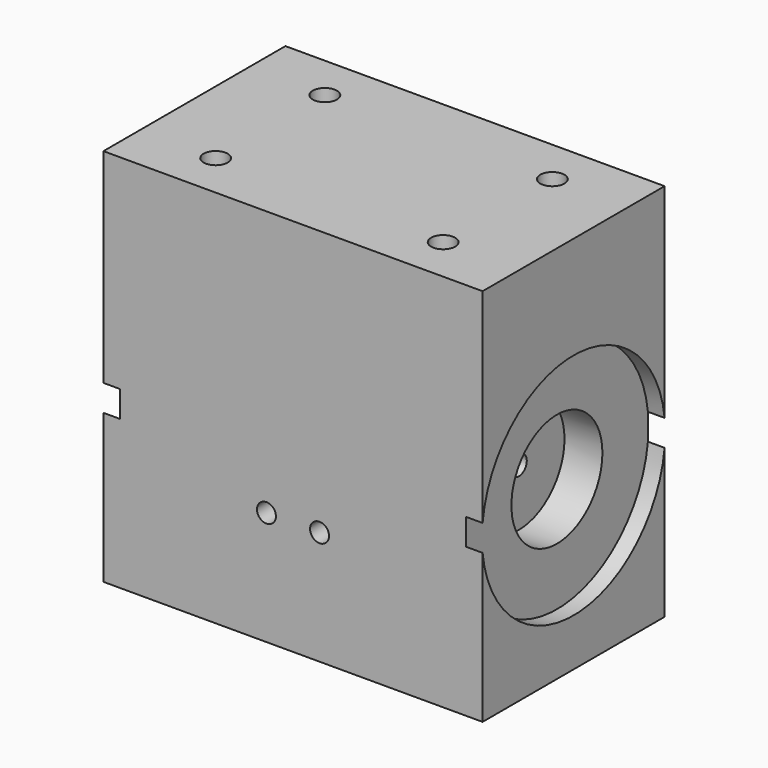
from build123d import *
from build123d import SkipClean  # not in build123d's __all__

# Parameters (mm, degrees)
F0_W      = 63.5
F0_H      = 38.1
F0_R      = 2.0193
F1_DEPTH  = 63.5
F2_DEPTH  = 25.4
F3_R      = 2.0193
F4_DEPTH  = 25.4
F5_R      = 1.5875
F6_DEPTH  = 19.05
F7_R      = 1.5875
F8_DEPTH  = 20.32
F9_R      = 1.63195
F10_DEPTH = 63.501
F9_R_2    = 9.525
F11_DEPTH = 9.144
F12_DEPTH = 2.794
F13_R     = 9.525
F13_R_2   = 1.63195
F14_DEPTH = 9.144
F15_DEPTH = 2.794


with BuildPart() as f1:
    # F0 (on Top) → F1 (new body)
    with BuildSketch(Plane.XY):
        Rectangle(F0_W, F0_H)
        with Locations((-24.13, -11.43)):
            Circle(F0_R, mode=Mode.SUBTRACT)
        with Locations((24.13, -11.43)):
            Circle(F0_R, mode=Mode.SUBTRACT)
        with Locations((-24.13, 11.43)):
            Circle(F0_R, mode=Mode.SUBTRACT)
        with Locations((24.13, 11.43)):
            Circle(F0_R, mode=Mode.SUBTRACT)
        with Locations((-24.13, 11.43)):
            Circle(F0_R)
        with Locations((24.13, 11.43)):
            Circle(F0_R)
        with Locations((24.13, -11.43)):
            Circle(F0_R)
        with Locations((-24.13, -11.43)):
            Circle(F0_R)
    extrude(amount=F1_DEPTH)

    # F0 (on Top) → F2 (cut)
    with BuildSketch(Plane.XY):
        with Locations((24.13, 11.43)):
            Circle(F0_R)
        with Locations((24.13, -11.43)):
            Circle(F0_R)
        with Locations((-24.13, 11.43)):
            Circle(F0_R)
        with Locations((-24.13, -11.43)):
            Circle(F0_R)
    extrude(amount=F2_DEPTH, mode=Mode.SUBTRACT)

    # F3 (on face) → F4 (cut)
    with BuildSketch(Plane.XY.offset(63.5)):
        with Locations((-19.05, 11.43)):
            Circle(F3_R)
        with Locations((-19.05, -11.43)):
            Circle(F3_R)
        with Locations((19.05, 11.43)):
            Circle(F3_R)
        with Locations((19.05, -11.43)):
            Circle(F3_R)
    extrude(amount=-F4_DEPTH, mode=Mode.SUBTRACT)

    # F5 (on face) → F6 (cut)
    with BuildSketch(Plane.XY):
        with Locations((-4.445, 0)):
            Circle(F5_R)
        with Locations((4.445, 0)):
            Circle(F5_R)
    extrude(amount=F6_DEPTH, mode=Mode.SUBTRACT)

    # F7 (on face) → F8 (cut)
    with BuildSketch(Plane.XZ.offset(19.05)):
        with Locations((-4.445, 19.05)):
            Circle(F7_R)
        with Locations((4.445, 19.05)):
            Circle(F7_R)
    with SkipClean():  # cleaning this boolean's faces spoils the solid; the shape is the same uncleaned
        extrude(amount=-F8_DEPTH, mode=Mode.SUBTRACT)

    # F9 (on face) → F10 (cut, through all)
    with BuildSketch(Plane.YZ.offset(31.75)):
        with Locations((0, 27.1272)):
            Circle(F9_R)
    with SkipClean():  # cleaning this boolean's faces spoils the solid; the shape is the same uncleaned
        extrude(amount=-F10_DEPTH, mode=Mode.SUBTRACT)

    # F9 (on face) → F11 (cut)
    with BuildSketch(Plane.YZ.offset(31.75)):
        with Locations((0, 27.1272)):
            Circle(F9_R_2)
        with Locations((0, 27.1272)):
            Circle(F9_R, mode=Mode.SUBTRACT)
    with SkipClean():  # cleaning this boolean's faces spoils the solid; the shape is the same uncleaned
        extrude(amount=-F11_DEPTH, mode=Mode.SUBTRACT)

    # F9 (on face) → F12 (cut)
    with BuildSketch(Plane.YZ.offset(31.75)):
        with BuildLine():
            Line((19.05, 24.9238323502), (19.05, 29.3305676498))
            ThreePointArc((19.05, 29.3305676498), (0, 46.3042), (-19.05, 29.3305676498))
            Line((-19.05, 29.3305676498), (-19.05, 24.9238323502))
            ThreePointArc((-19.05, 24.9238323502), (0, 7.9502), (19.05, 24.9238323502))
        make_face()
        with Locations((0, 27.1272)):
            Circle(F9_R_2, mode=Mode.SUBTRACT)
    with SkipClean():  # cleaning this boolean's faces spoils the solid; the shape is the same uncleaned
        extrude(amount=-F12_DEPTH, mode=Mode.SUBTRACT)

    # F13 (on face) → F14 (cut)
    with BuildSketch(Plane(origin=(-31.75, 0, 0), x_dir=(0, -1, 0), z_dir=(-1, 0, 0))):
        with Locations((0, 27.1272)):
            Circle(F13_R)
        with Locations((0, 27.1272)):
            Circle(F13_R_2, mode=Mode.SUBTRACT)
    with SkipClean():  # cleaning this boolean's faces spoils the solid; the shape is the same uncleaned
        extrude(amount=-F14_DEPTH, mode=Mode.SUBTRACT)

    # F13 (on face) → F15 (cut)
    with BuildSketch(Plane(origin=(-31.75, 0, 0), x_dir=(0, -1, 0), z_dir=(-1, 0, 0))):
        with BuildLine():
            Line((19.05, 24.9238323502), (19.05, 29.3305676498))
            ThreePointArc((19.05, 29.3305676498), (0, 46.3042), (-19.05, 29.3305676498))
            Line((-19.05, 29.3305676498), (-19.05, 24.9238323502))
            ThreePointArc((-19.05, 24.9238323502), (0, 7.9502), (19.05, 24.9238323502))
        make_face()
        with Locations((0, 27.1272)):
            Circle(F13_R, mode=Mode.SUBTRACT)
    with SkipClean():  # cleaning this boolean's faces spoils the solid; the shape is the same uncleaned
        extrude(amount=-F15_DEPTH, mode=Mode.SUBTRACT)


solid = f1.part
